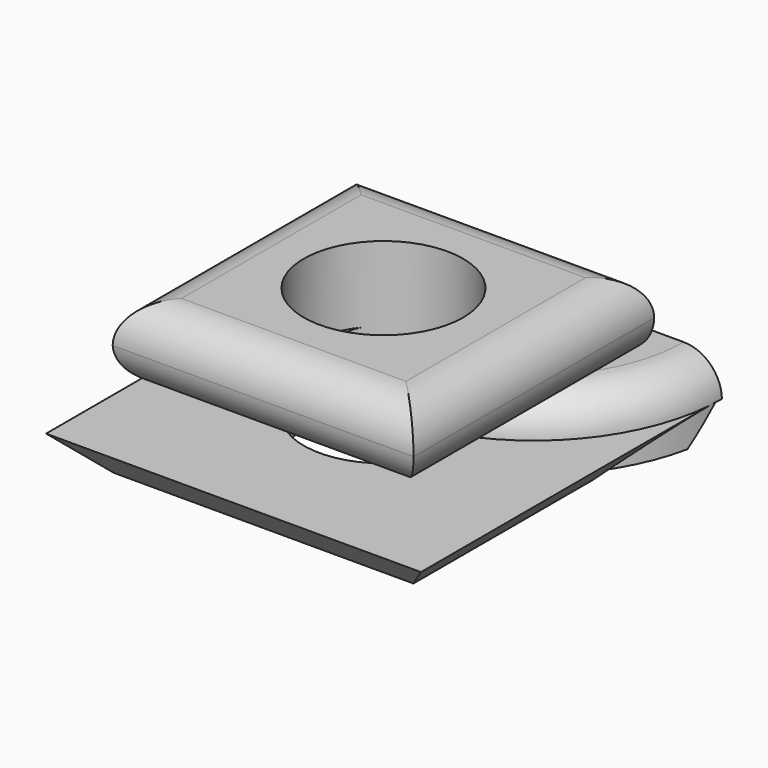
from build123d import *

# Parameters (mm, degrees)
F1_DEPTH      = 5
F2_DEPTH      = 5
F3_T2_ANGLE   = 238.3061287116
F4_DEPTH      = 4
F5_T1_DEPTH   = 85.2732038629
F5_T3_DEPTH   = 76.1282991577
F5_2_T1_DEPTH = 76.1270392372
F7_W          = 40
F7_H          = 40
F8_DEPTH      = 10
F9_R          = 5.08
F10_T1_DEPTH  = 65.3873984488
F10_T3_DEPTH  = 65.3873984488
F12_R         = 10.5941406936
F13_DEPTH     = 76.2


# Not quite as in the source:
# - a fillet or chamfer that OpenCascade refuses, or shapes differently, is made with other operations: its cross-section is extruded or revolved along the edge and cut away or added


with BuildPart() as f1:
    # F0 (on Top) → F1 (new body)
    with BuildSketch(Plane.XY):
        with BuildLine():
            Line((-25, -25), (25, -25))
            Line((25, -25), (25, 25))
            ThreePointArc((25, 25), (0, 0), (-25, 25))
            Line((-25, 25), (-25, -25))
        make_face()
    extrude(amount=-F1_DEPTH)

    # F5: chamfer of 5.08 on 3 edges, made by hand

    # F5_s2 → F5_t1 (cut)
    with BuildSketch(Plane.XZ.offset(-47.2090542841)):
        Polygon((-25, 0.08), (-19.92, -5), (-25, -5), align=None)
        Polygon((25, 0.08), (19.92, -5), (25, -5), align=None)
    extrude(amount=F5_T1_DEPTH, mode=Mode.SUBTRACT)

    # F5_s4 → F5_t3 (cut)
    with BuildSketch(Plane.YZ.offset(-38.0641495789)):
        Polygon((-25, 0.08), (-19.92, -5), (-25, -5), align=None)
    extrude(amount=F5_T3_DEPTH, mode=Mode.SUBTRACT)


with BuildPart() as f2:
    # F0 (on Top) → F2 (new body)
    with BuildSketch(Plane.XY):
        with BuildLine():
            ThreePointArc((-25, 25), (0, 0), (25, 25))
            Line((25, 25), (-25, 25))
        make_face()
    extrude(amount=F2_DEPTH)

    # F3: fillet of radius 5.08 on 1 edges, made by hand

    # F3_s1 → F3_t2 (revolve, cut)
    with BuildSketch(Plane(origin=(10.6358414033, 19.0672580005, 0), x_dir=(0, 0, 1), z_dir=(0.4871444139, 0.87332143, 0))):
        with BuildLine():
            ThreePointArc((-0.08, -37.1786103472), (3.5121024484, -35.6907127956), (5, -32.0986103472))
            Line((5, -32.0986103472), (5, -37.1786103472))
            Line((5, -37.1786103472), (-0.08, -37.1786103472))
        make_face()
    revolve(axis=Axis((0, 25, 5), (0, 0, 1)), revolution_arc=F3_T2_ANGLE, mode=Mode.SUBTRACT)


with BuildPart() as f4:
    # F4 (new): a face of the model
    f4_faces = [f2.part.faces().sort_by_distance(p)[0] for p in [
        (0, 14.389937824, 0),
    ]]
    extrude(f4_faces, amount=F4_DEPTH)

    # F5#2: chamfer of 5.08 on 1 edges, made by hand

    # F5_2_s2 → F5_2_t1 (cut)
    with BuildSketch(Plane.YZ.offset(-38.0635196186)):
        Polygon((25, 1.08), (19.92, -4), (25, -4), align=None)
    extrude(amount=F5_2_T1_DEPTH, mode=Mode.SUBTRACT)


with BuildPart() as f2_1:
    add(f2.part)

    # F7 (on offset) → F8 (join)
    with BuildSketch(Plane.XY.offset(5)):
        Rectangle(F7_W, F7_H)
    extrude(amount=F8_DEPTH)

    # F9
    f9_edges = [f2_1.edges().sort_by_distance(p)[0] for p in [
        (-20, 0, 15),
        (0, 20, 15),
        (20, 0, 15),
        (0, -20, 15),
    ]]
    fillet(f9_edges, radius=F9_R)

    # F10: fillet of radius 5.08 on 3 edges, made by hand

    # F10_s2 → F10_t1 (cut)
    with BuildSketch(Plane.XZ.offset(-32.6936992244)):
        with BuildLine():
            ThreePointArc((20, 9.92), (18.4576016389, 6.4317675513), (14.9225203102, 5))
            Line((14.9225203102, 5), (20, 5))
            Line((20, 5), (20, 9.92))
        make_face()
        with BuildLine():
            ThreePointArc((-14.9225203102, 5), (-18.4576016389, 6.4317675513), (-20, 9.92))
            Line((-20, 9.92), (-20, 5))
            Line((-20, 5), (-14.9225203102, 5))
        make_face()
    extrude(amount=F10_T1_DEPTH, mode=Mode.SUBTRACT)

    # F10_s4 → F10_t3 (cut)
    with BuildSketch(Plane.YZ.offset(-32.6936992244)):
        with BuildLine():
            ThreePointArc((-14.9225203102, 5), (-18.4576016389, 6.4317675513), (-20, 9.92))
            Line((-20, 9.92), (-20, 5))
            Line((-20, 5), (-14.9225203102, 5))
        make_face()
    extrude(amount=F10_T3_DEPTH, mode=Mode.SUBTRACT)


with BuildPart() as f13_tool:
    # F12 (on offset) → F13 (new body)
    with BuildSketch(Plane.XY.offset(15)):
        Circle(F12_R)
    extrude(amount=-F13_DEPTH)


with BuildPart() as f1_1:
    add(f1.part)

    # F13: cut by f13_tool
    add(f13_tool.part, mode=Mode.SUBTRACT)


with BuildPart() as f2_2:
    add(f2_1.part)

    # F13: cut by f13_tool
    add(f13_tool.part, mode=Mode.SUBTRACT)


with BuildPart() as f4_1:
    add(f4.part)

    # F13: cut by f13_tool
    add(f13_tool.part, mode=Mode.SUBTRACT)


solid = Compound([f1_1.part, f2_2.part, f4_1.part])
